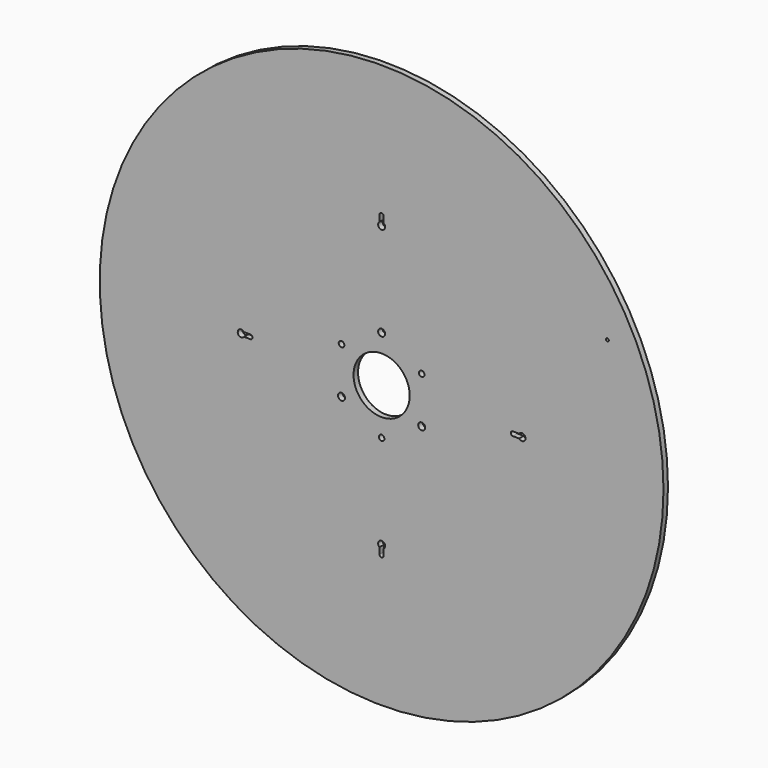
from build123d import *

# Parameters (mm, degrees)
F0_R            = 1004.05
F0_R_2          = 100
F1_DEPTH        = 20
F2_D            = 25
F2_DEPTH        = 28
F2_TIP          = 7.5107577378
F2_COPIES_COUNT = 3
F3_D            = 20
F3_DEPTH        = 28
F3_TIP          = 6.0086061903
F3_COPIES_COUNT = 3
F4_D            = 10
F4_DEPTH        = 28
F4_TIP          = 3.0043030951


# Not quite as in the source:
# - a pattern or mirror of a feature is missing from the dataset's text; its kind, count and spacing are read off the source's solid


with BuildPart() as f1:
    # F0 (on Front) → F1 (new body)
    with BuildSketch(Plane.XZ):
        Circle(F0_R)
        with BuildLine():
            ThreePointArc((12.5, -500), (11.1803398875, -505.5901699437), (7.5, -510))
            Line((7.5, -510), (7.5, -532.5))
            ThreePointArc((7.5, -532.5), (5.3033008589, -537.8033008589), (0, -540))
            ThreePointArc((0, -540), (-5.3033008589, -537.8033008589), (-7.5, -532.5))
            Line((-7.5, -532.5), (-7.5, -510))
            ThreePointArc((-7.5, -510), (-5.5901699437, -488.8196601125), (12.5, -500))
        make_face(mode=Mode.SUBTRACT)
        with BuildLine():
            ThreePointArc((-490, -7.5), (-512.5, 0), (-490, 7.5))
            Line((-490, 7.5), (-467.5, 7.5))
            ThreePointArc((-467.5, 7.5), (-462.1966991411, 5.3033008589), (-460, 0))
            ThreePointArc((-460, 0), (-462.1966991411, -5.3033008589), (-467.5, -7.5))
            Line((-467.5, -7.5), (-490, -7.5))
        make_face(mode=Mode.SUBTRACT)
        Circle(F0_R_2, mode=Mode.SUBTRACT)
        with BuildLine():
            ThreePointArc((512.5, 0), (503.9528470752, -11.8585412256), (490, -7.5))
            Line((490, -7.5), (467.5, -7.5))
            ThreePointArc((467.5, -7.5), (462.1966991411, -5.3033008589), (460, 0))
            ThreePointArc((460, 0), (462.1966991411, 5.3033008589), (467.5, 7.5))
            Line((467.5, 7.5), (490, 7.5))
            ThreePointArc((490, 7.5), (503.9528470752, 11.8585412256), (512.5, 0))
        make_face(mode=Mode.SUBTRACT)
        with BuildLine():
            ThreePointArc((7.5, 510), (11.1803398875, 505.5901699437), (12.5, 500))
            ThreePointArc((12.5, 500), (-5.5901699437, 488.8196601125), (-7.5, 510))
            Line((-7.5, 510), (-7.5, 532.5))
            ThreePointArc((-7.5, 532.5), (-5.3033008589, 537.8033008589), (0, 540))
            ThreePointArc((0, 540), (5.3033008589, 537.8033008589), (7.5, 532.5))
            Line((7.5, 532.5), (7.5, 510))
        make_face(mode=Mode.SUBTRACT)
    extrude(amount=-F1_DEPTH)

    # F2
    with Locations(Plane.XZ):
        with Locations((0, 165)):
            f2 = Hole(F2_D / 2, depth=F2_DEPTH)
            with Locations((0, 0, -(F2_DEPTH + F2_TIP / 2))):  # 118° drill point
                Cone(0, F2_D / 2, F2_TIP, mode=Mode.SUBTRACT)

    # F2_copies: F2 ×3 about axis
    f2_copies_axis = Axis((0, 0, 0), (0, 1, 0))
    for i in range(1, F2_COPIES_COUNT):
        add(f2.rotate(f2_copies_axis, i * 360 / F2_COPIES_COUNT), mode=Mode.SUBTRACT)

    # F3
    with Locations(Plane.XZ):
        with Locations((142.8941916244, 82.5)):
            f3 = Hole(F3_D / 2, depth=F3_DEPTH)
            with Locations((0, 0, -(F3_DEPTH + F3_TIP / 2))):  # 118° drill point
                Cone(0, F3_D / 2, F3_TIP, mode=Mode.SUBTRACT)

    # F3_copies: F3 ×3 about axis
    f3_copies_axis = Axis((0, 0, 0), (0, 1, 0))
    for i in range(1, F3_COPIES_COUNT):
        add(f3.rotate(f3_copies_axis, i * 360 / F3_COPIES_COUNT), mode=Mode.SUBTRACT)

    # F4
    with Locations(Plane.XZ):
        with Locations((804.2584775463, 403.9409626355)):
            Hole(F4_D / 2, depth=F4_DEPTH)
            with Locations((0, 0, -(F4_DEPTH + F4_TIP / 2))):  # 118° drill point
                Cone(0, F4_D / 2, F4_TIP, mode=Mode.SUBTRACT)


solid = f1.part
